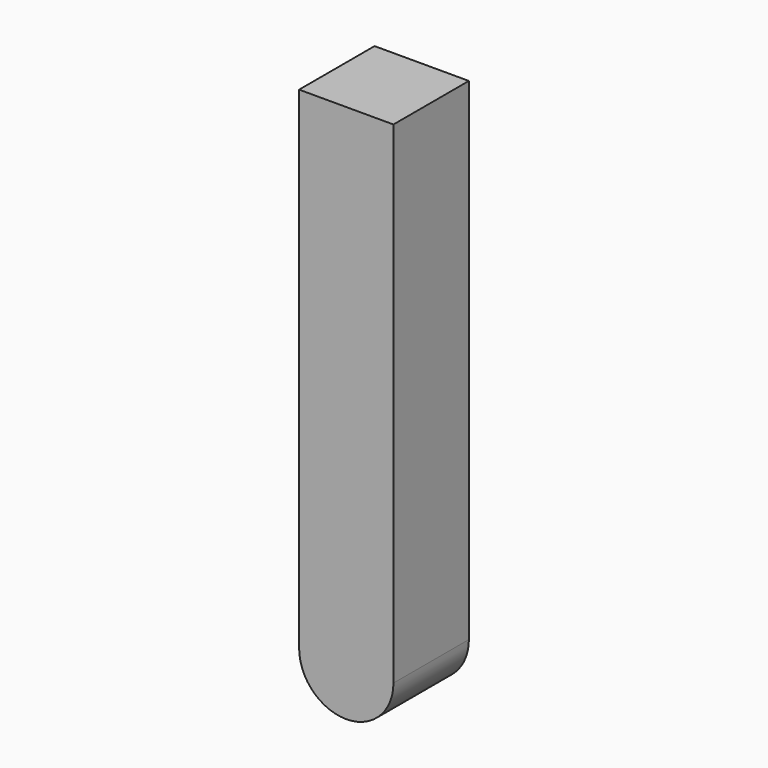
from build123d import *

# Parameters (mm, degrees)
F0_W     = 7
F0_H     = 40
F1_DEPTH = 7
F2_R     = 3.49999


# Not quite as in the source:
# - a fillet or chamfer is up to 0.001 mm smaller than in the source, because OpenCascade refuses the exact size


with BuildPart() as f1:
    # F0 (on Front) → F1 (new body)
    with BuildSketch(Plane.XZ):
        Rectangle(F0_W, F0_H)
    extrude(amount=F1_DEPTH)

    # F2 (radius 3.5 in the source; OpenCascade refuses exactly that, so slightly less here)
    f2_edges = [f1.edges().sort_by_distance(p)[0] for p in [
        (3.5, -3.5, -20),
        (-3.5, -3.5, -20),
    ]]
    fillet(f2_edges, radius=F2_R)


solid = f1.part
